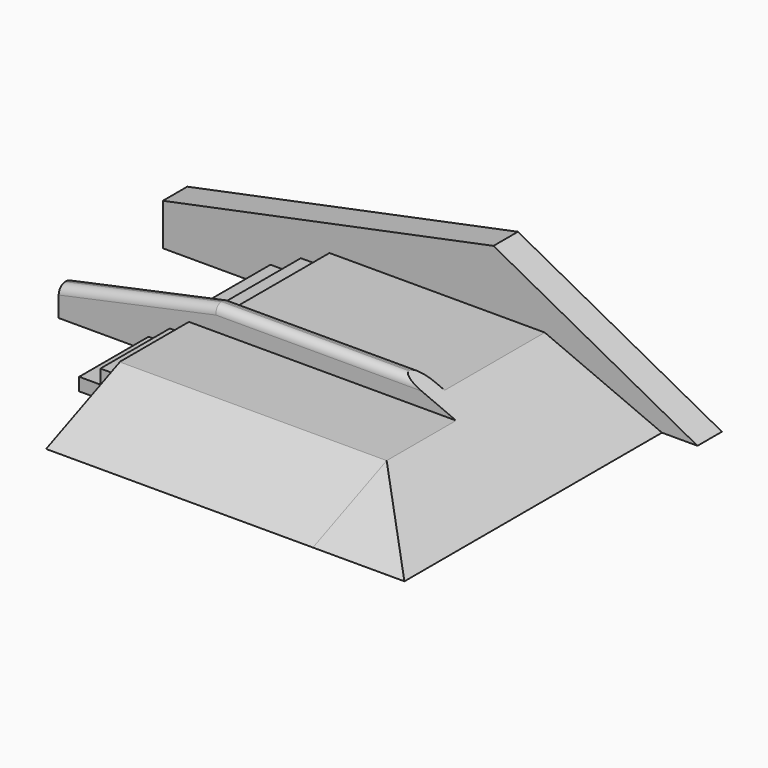
from build123d import *

# Parameters (mm, degrees)
F1_DEPTH     = 113.387234509
F3_DEPTH     = 464.7335410118
F5_DEPTH     = 66.4555206895
F6_R         = 30.48
F8_DEPTH     = 322.3102986813
F10_DEPTH    = 342.2025442123
F12_DEPTH    = 991.1689758301
F13_T4_DEPTH = 1291.048119331


# Not quite as in the source:
# - a fillet or chamfer that OpenCascade refuses, or shapes differently, is made with other operations: its cross-section is extruded or revolved along the edge and cut away or added


with BuildPart() as f1:
    # F0 (on Front) → F1 (new body)
    with BuildSketch(Plane.XZ):
        Polygon((-915.6464338303, -243.6540126801), (1070.1038837433, -243.6540126801), (312.4090433121, 163.7299656868), (-915.6464338303, -88.1789922714), align=None)
    extrude(amount=-F1_DEPTH)

    # F2 (on face) → F3 (join)
    with BuildSketch(Plane.XZ):
        Polygon((-516.0537958145, -243.6540126801), (938.1332397461, -243.6540126801), (502.8445720673, -57.6961040497), (-296.7971563339, -57.6961040497), (-296.7971563339, -109.2859506607), (-403.2011032104, -109.2859506607), (-403.2011032104, -167.32442379), (-516.0537958145, -167.32442379), align=None)
    extrude(amount=F3_DEPTH)

    # F4 (on face) → F5 (join)
    with BuildSketch(Plane.XZ.offset(464.7335410118)):
        Polygon((528.1958580017, -243.6540126801), (938.1332397461, -243.6540126801), (398.7933658153, -13.2448096747), (-296.7971563339, -13.2448096747), (-877.5278925896, -136.8308067322), (-877.5278925896, -243.4085607529), align=None)
    extrude(amount=F5_DEPTH)

    # F6
    f6_edges = [f1.edges().sort_by_distance(p)[0] for p in [
        (50.998105, -464.733541, -13.24481),
        (50.998105, -531.189062, -13.24481),
        (-587.162524, -531.189062, -75.037808),
        (-587.162524, -464.733541, -75.037808),
    ]]
    fillet(f6_edges, radius=F6_R)

    # F7 (on face) → F8 (join)
    with BuildSketch(Plane.XZ.offset(531.1890617013)):
        Polygon((-543.689250946, -243.4668519626), (938.1332397461, -243.6540126801), (598.4011143715, -98.5184274462), (-393.8011527061, -98.5184274462), (-393.8011527061, -143.1138366461), (-464.6941423416, -143.1138366461), (-464.6941423416, -195.7771629095), (-543.689250946, -195.7771629095), align=None)
    extrude(amount=F8_DEPTH)

    # F9 (on face) → F10 (join)
    with BuildSketch(Plane.XZ.offset(853.4993603826)):
        Polygon((938.1332397461, -243.6540126801), (598.4011143715, -98.5184274462), (598.4011143715, -243.6111030139), align=None)
    extrude(amount=F10_DEPTH)

    # F11 (on face) → F12 (join)
    with BuildSketch(Plane(origin=(598.4011143715, 0, 0), x_dir=(0, -1, 0), z_dir=(-1, 0, 0))):
        Polygon((853.4993603826, -98.5184274462), (853.4993603826, -243.6111030139), (1195.7019045949, -243.6111030139), align=None)
    extrude(amount=F12_DEPTH)

    # F13: chamfer of 254 x 368.3 on 1 edges, made by hand


with BuildPart() as f13_tool2:
    # F13_s3 → F13_t4 (new body)
    with BuildSketch(Plane.XZ.offset(853.4993603826)):
        Polygon((937.089450141, -243.2080995506), (598.4011143715, -352.5184274462), (598.4011143715, -98.5184274462), align=None)
    extrude(amount=F13_T4_DEPTH)

    split(bisect_by=Plane(origin=(0, -94.6492992071, 223.2313303883), x_dir=(1, 0, 0), z_dir=(0, -0.3903579472, 0.9206631703)), keep=Keep.TOP)


with BuildPart() as f1_1:
    add(f1.part)

    # F13_t1: cut F13_tool2
    add(f13_tool2.part, mode=Mode.SUBTRACT)


solid = f1_1.part
